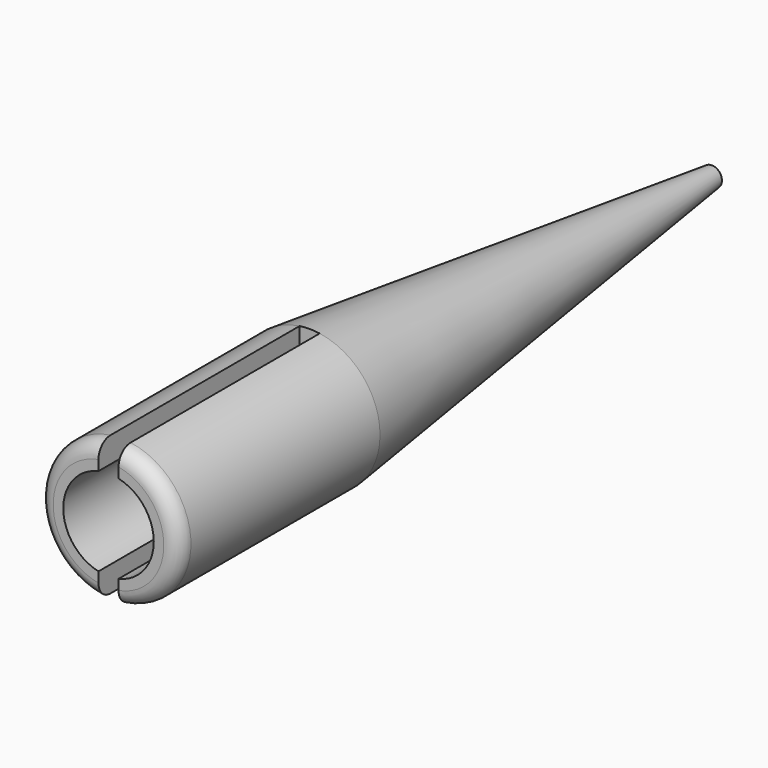
from build123d import *

# Parameters (mm, degrees)
F0_R      = 7
F1_DEPTH  = 25
F3_R      = 1
F1_FACE_R = 7
F5_T      = -2.5
F6_R      = 1.5
F8_W      = 2
F8_H      = 21.4920276658
F9_DEPTH  = 25


# Not quite as in the source:
# - a shell that OpenCascade refuses in one call is made with other operations: the cavity is built on its own and cut out
# - a feature names something its author has since deleted; it is built from what else it names


with BuildPart() as f1:
    # F0 (on Front) → F1 (new body)
    with BuildSketch(Plane.XZ):
        Circle(F0_R)
    extrude(amount=F1_DEPTH)

    # F3 (on offset) → F4 section 0
    with BuildSketch(Plane.XZ.offset(-50)):
        Circle(F3_R)
    # F1_face (on face) → F4 section 1
    with BuildSketch(Plane(origin=(0, 0, 0), x_dir=(1, 0, 0), z_dir=(0, 1, 0))):
        Circle(F1_FACE_R)
    loft()

    # F5: a shell. OpenCascade refuses it in one call, so the cavity is built on its own and cut out:
    # the body offset inwards by the wall thickness, plus a prism from it out through each open face.
    f5_core = offset(f1.part, amount=F5_T, mode=Mode.PRIVATE)
    f5_exits = [f5_core.faces().sort_by_distance(p)[0] for p in [
        (0, -22.5, 0),
    ]]
    add(f5_core, mode=Mode.SUBTRACT)
    extrude(f5_exits, amount=-F5_T, mode=Mode.SUBTRACT)

    # F6
    f6_edges = [f1.edges().sort_by_distance(p)[0] for p in [
        (-7, -25, 0),
    ]]
    fillet(f6_edges, radius=F6_R)

    # F8 (on offset) → F9 (cut)
    with BuildSketch(Plane.XZ.offset(25)):
        Rectangle(F8_W, F8_H)
    extrude(amount=-F9_DEPTH, mode=Mode.SUBTRACT)


solid = f1.part
